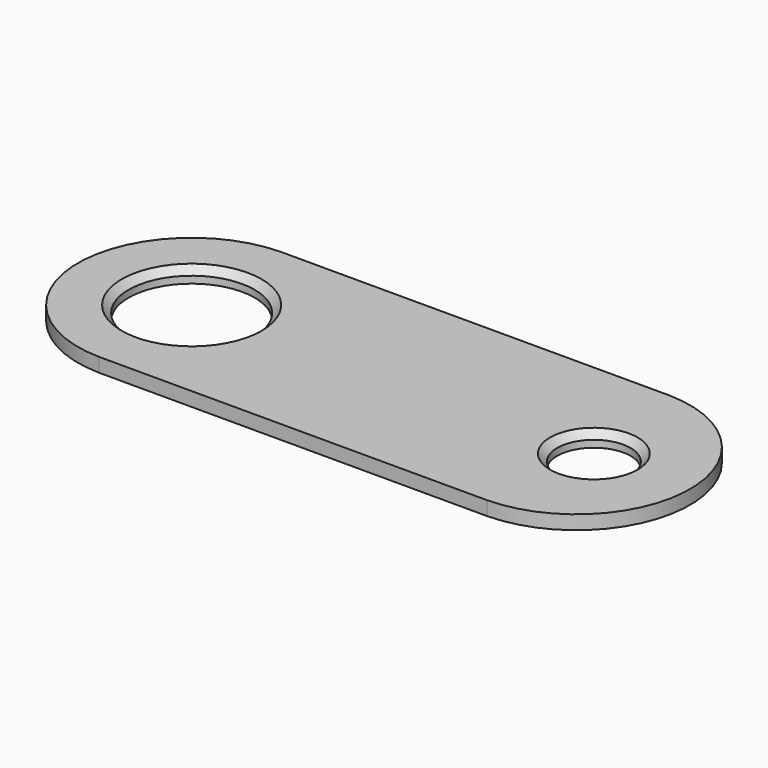
from build123d import *

# Parameters (mm, degrees)
F0_R     = 18
F0_R_2   = 10.5
F1_DEPTH = 4
F2_SIZE  = 2


# Not quite as in the source:
# - a feature names something its author has since deleted; it is built from what else it names


with BuildPart() as f1:
    # F0 (on Top) → F1 (new body)
    with BuildSketch(Plane.XY):
        with BuildLine():
            ThreePointArc((-55.5, 32.5), (-87.5, 0), (-55.5, -32.5))
            Line((-55.5, -32.5), (55.5, -32.5))
            ThreePointArc((55.5, -32.5), (87.5, 0), (55.5, 32.5))
            Line((55.5, 32.5), (-55.5, 32.5))
        make_face()
        with Locations((-55, 0)):
            Circle(F0_R, mode=Mode.SUBTRACT)
        with Locations((60, 0)):
            Circle(F0_R_2, mode=Mode.SUBTRACT)
    extrude(amount=F1_DEPTH)

    # F2
    f2_edges = [f1.edges().sort_by_distance(p)[0] for p in [
        (-73, 0, 4),
        (49.5, 0, 4),
    ]]
    chamfer(f2_edges, length=F2_SIZE)


solid = f1.part
